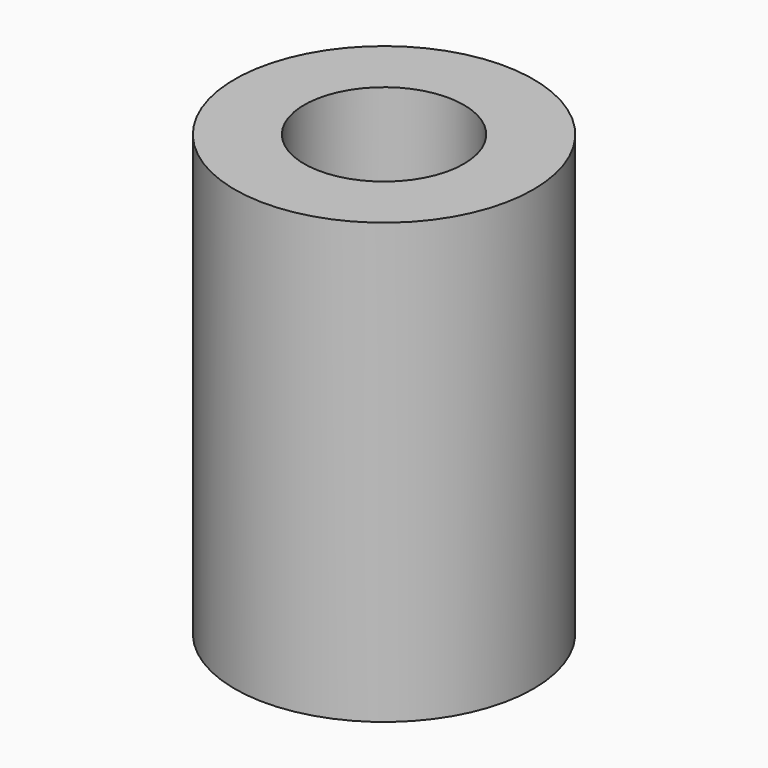
from build123d import *

# Parameters (mm, degrees)
F0_R     = 9.1481324812
F0_R_2   = 4.8908401844
F2_DEPTH = 25.4
F3_R     = 9.1481324812
F3_R_2   = 4.5098401844
F4_DEPTH = 1.524


# Not quite as in the source:
# - the program builds the solid bodies; features that only make, move or delete a surface that nothing else refers to are left out


with BuildPart() as f2:
    # F0 (on Top) → F2 (new body)
    with BuildSketch(Plane.XY):
        Circle(F0_R)
        Circle(F0_R_2, mode=Mode.SUBTRACT)
    extrude(amount=F2_DEPTH)

    # F3 (on face) → F4 (join)
    with BuildSketch(Plane(origin=(0, 0, 0), x_dir=(1, 0, 0), z_dir=(0, 0, -1))):
        Circle(F3_R)
        Circle(F3_R_2, mode=Mode.SUBTRACT)
    extrude(amount=F4_DEPTH)


solid = f2.part
